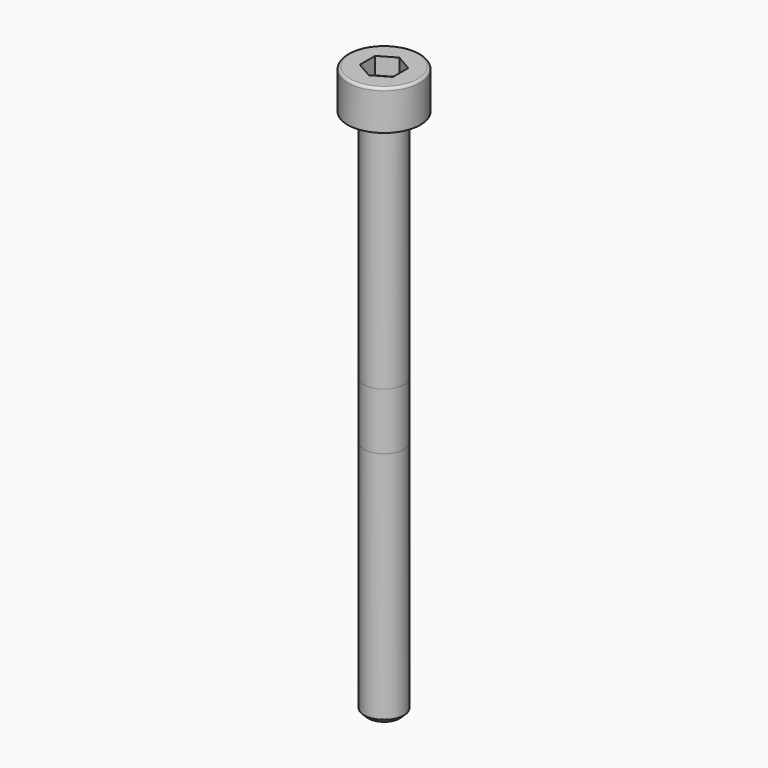
from build123d import *

# Parameters (mm, degrees)
F4_DEPTH = 1.3


with BuildPart() as f2:
    # F1 (on Front) → F2 (revolve)
    with BuildSketch(Plane.XZ):
        with BuildLine():
            Line((2.55, 3), (0, 3))
            Line((0, 3), (0, 0))
            Line((0, 0), (2.75, 0))
            Line((2.75, 0), (2.75, 2.8))
            ThreePointArc((2.75, 2.8), (2.6914213562, 2.9414213562), (2.55, 3))
        make_face()
    revolve(axis=Axis((0, 0, 1.5), (0, 0, 1)))

    # F3 (on face) → F4 (cut)
    with BuildSketch(Plane.XY.offset(3)):
        Polygon((1.25, -0.7216878365), (1.25, 0.7216878365), (0, 1.443375673), (-1.25, 0.7216878365), (-1.25, -0.7216878365), (0, -1.443375673), align=None)
    extrude(amount=-F4_DEPTH, mode=Mode.SUBTRACT)


with BuildPart() as f5_1:
    # F5: copy of F2
    add(f2.part)

    # F6 (on Front) → F7 (revolve)
    with BuildSketch(Plane.XZ):
        Polygon((1.5, 0), (0, 0), (0, -8), (1.2, -8), (1.5, -7.7), align=None)
    revolve(axis=Axis((0, 0, -4), (0, 0, -1)))


with BuildPart() as f8_1:
    # F8: copy of F2
    add(f2.part)

    # F9 (on Front) → F10 (revolve)
    with BuildSketch(Plane.XZ):
        Polygon((1.5, 0), (0, 0), (0, -10), (1.2, -10), (1.5, -9.7), align=None)
    revolve(axis=Axis((0, 0, -5), (0, 0, -1)))


with BuildPart() as f11_1:
    # F11: copy of F2
    add(f2.part)

    # F12 (on Front) → F13 (revolve)
    with BuildSketch(Plane.XZ):
        Polygon((1.5, 0), (0, 0), (0, -30), (1.2, -30), (1.5, -29.7), align=None)
    revolve(axis=Axis((0, 0, -15), (0, 0, -1)))


with BuildPart() as f14_1:
    # F14: copy of F2
    add(f2.part)

    # F15 (on Front) → F16 (revolve)
    with BuildSketch(Plane.XZ):
        Polygon((1.5, 0), (0, 0), (0, -40), (1.2, -40), (1.5, -39.7), (1.5, -22.0115470054), (1.48, -22), (1.5, -22), align=None)
    revolve(axis=Axis((0, 0, -20), (0, 0, -1)))


with BuildPart() as f17_1:
    # F17: copy of F2
    add(f2.part)

    # F18 (on Front) → F19 (revolve)
    with BuildSketch(Plane.XZ):
        Polygon((1.5, 0), (0, 0), (0, -6), (1.2, -6), (1.5, -5.7), align=None)
    revolve(axis=Axis((0, 0, -3), (0, 0, -1)))


with BuildPart() as f20_1:
    # F20: copy of F2
    add(f2.part)

    # F21 (on Front) → F22 (revolve)
    with BuildSketch(Plane.XZ):
        Polygon((1.5, 0), (0, 0), (0, -16), (1.2, -16), (1.5, -15.7), align=None)
    revolve(axis=Axis((0, 0, -8), (0, 0, 1)))


with BuildPart() as f23_1:
    # F23: copy of F2
    add(f2.part)

    # F24 (on Front) → F25 (revolve)
    with BuildSketch(Plane.XZ):
        Polygon((1.5, 0), (0, 0), (0, -12), (1.2, -12), (1.5, -11.7), align=None)
    revolve(axis=Axis((0, 0, -6), (0, 0, 1)))


with BuildPart() as f26_1:
    # F26: copy of F2
    add(f2.part)

    # F27 (on Front) → F28 (revolve)
    with BuildSketch(Plane.XZ):
        Polygon((1.5, 0), (0, 0), (0, -18), (1.2, -18), (1.5, -17.7), align=None)
    revolve(axis=Axis((0, 0, -9), (0, 0, 1)))


solid = Compound([f2.part, f5_1.part, f8_1.part, f11_1.part, f14_1.part, f17_1.part, f20_1.part, f23_1.part, f26_1.part])
